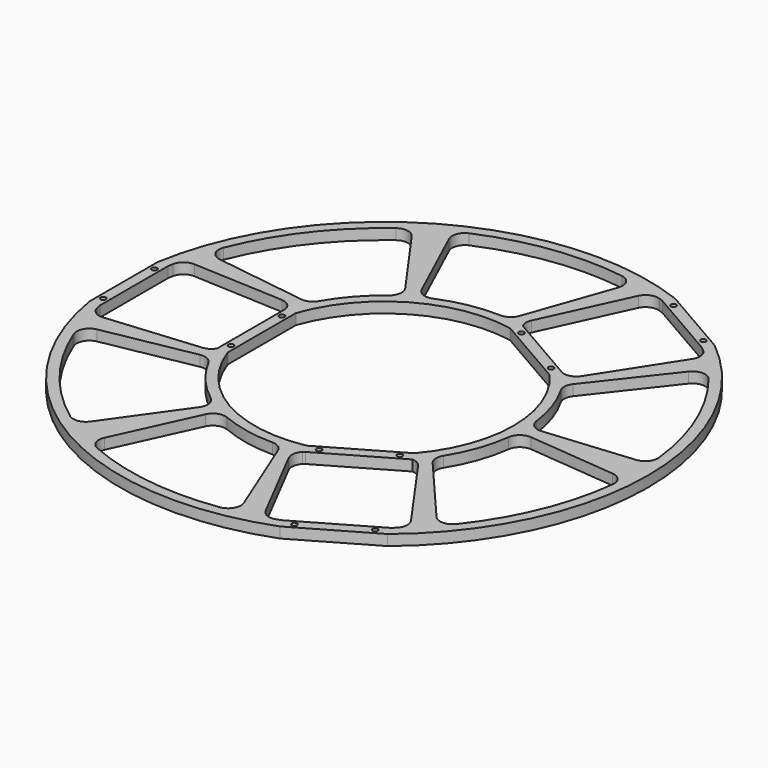
from build123d import *

# Parameters (mm, degrees)
F0_W        = 6.35
F0_H        = 50.8
F0_R        = 1.5875
F1_DEPTH    = 6.35
F4_DEPTH    = 6.35
F5_T1_DEPTH = 6.35
F6_R        = 5.08
F7_COUNT    = 3


# Not quite as in the source:
# - a fillet or chamfer that OpenCascade refuses, or shapes differently, is made with other operations: its cross-section is extruded or revolved along the edge and cut away or added
# - a feature of the source that left no trace in its solid (it failed there, or was rolled back) is left out


with BuildPart() as f1:
    # F0 (on Top) → F1 (new body)
    with BuildSketch(Plane.XY):
        with Locations((-76.2, 0)):
            Rectangle(F0_W, F0_H)
        with Locations((-76.2, -19.05)):
            Circle(F0_R, mode=Mode.SUBTRACT)
        with Locations((-76.2, 19.05)):
            Circle(F0_R, mode=Mode.SUBTRACT)
    extrude(amount=F1_DEPTH)



with BuildPart() as f1b:
    # F0 (on Top) → F1, piece 2 (new body)
    with BuildSketch(Plane.XY):
        with Locations((-152.4, 0)):
            Rectangle(F0_W, F0_H)
        with Locations((-152.4, -19.05)):
            Circle(F0_R, mode=Mode.SUBTRACT)
        with Locations((-152.4, 19.05)):
            Circle(F0_R, mode=Mode.SUBTRACT)
    extrude(amount=F1_DEPTH)


with BuildPart() as f1_1:
    add(f1.part)

    add(f1b.part)  # F4 merges F1b
    # F3 (on Top) → F4 (join)
    with BuildSketch(Plane.XY):
        with BuildLine():
            ThreePointArc((31.2797741547, 148.1041402319), (37.4651836805, 146.6615854162), (43.584633363, 144.9608235339))
            ThreePointArc((43.584633363, 144.9608235339), (48.1238684074, 143.5177825724), (52.6154547439, 141.9326408797))
            Line((52.6154547439, 141.9326408797), (55.7904547439, 147.4319021938))
            ThreePointArc((55.7904547439, 147.4319021938), (-78.8174165794, 136.5157700368), (-155.575, 25.4))
            Line((-155.575, 25.4), (-149.225, 25.4))
            ThreePointArc((-149.225, 25.4), (-148.3519798062, 30.0823987171), (-147.3320724153, 34.7350120599))
            ThreePointArc((-147.3320724153, 34.7350120599), (-145.7452505699, 40.8849918834), (-143.9018349238, 46.9629910733))
            ThreePointArc((-143.9018349238, 46.9629910733), (-120.5170928624, 91.5908890283), (-83.7806024253, 126.0716910423))
            ThreePointArc((-83.7806024253, 126.0716910423), (-75.6856337507, 131.0913630593), (-67.2909859281, 135.5919755658))
            ThreePointArc((-67.2909859281, 135.5919755658), (-19.0614902225, 150.1663085232), (31.2797741547, 148.1041402319))
        make_face()
        with BuildLine():
            ThreePointArc((8.2856324479, 82.9270698864), (11.4388872215, 82.551211282), (14.5755338083, 82.0554960938))
            Line((14.5755338083, 82.0554960938), (43.584633363, 144.9608235339))
            ThreePointArc((43.584633363, 144.9608235339), (37.4651836805, 146.6615854162), (31.2797741547, 148.1041402319))
            Line((31.2797741547, 148.1041402319), (8.2856324479, 82.9270698864))
        make_face()
        with BuildLine():
            ThreePointArc((-44.3888773768, 70.534943044), (-41.6699850762, 72.1745313026), (-38.8906138422, 73.7093669758))
            Line((-38.8906138422, 73.7093669758), (-67.2909859281, 135.5919755658))
            ThreePointArc((-67.2909859281, 135.5919755658), (-75.6856337507, 131.0913630593), (-83.7806024253, 126.0716910423))
            Line((-83.7806024253, 126.0716910423), (-44.3888773768, 70.534943044))
        make_face()
        with BuildLine():
            Line((-147.3320724153, 34.7350120599), (-77.2106727023, 31.3697728054))
            ThreePointArc((-77.2106727023, 31.3697728054), (-75.9595282254, 34.2884921917), (-74.5980976675, 37.1574279168))
            Line((-74.5980976675, 37.1574279168), (-143.9018349238, 46.9629910733))
            ThreePointArc((-143.9018349238, 46.9629910733), (-145.7452505699, 40.8849918834), (-147.3320724153, 34.7350120599))
        make_face()
        with BuildLine():
            ThreePointArc((-73.025, 25.4), (-38.6581512265, 66.957882051), (14.5154547439, 75.9415051114))
            Line((14.5154547439, 75.9415051114), (17.6904547439, 81.4407664254))
            ThreePointArc((17.6904547439, 81.4407664254), (16.1359219586, 81.762966235), (14.5755338083, 82.0554960938))
            ThreePointArc((14.5755338083, 82.0554960938), (11.4388872215, 82.551211282), (8.2856324479, 82.9270698864))
            ThreePointArc((8.2856324479, 82.9270698864), (-15.9814809475, 81.7932936843), (-38.8906138422, 73.7093669758))
            ThreePointArc((-38.8906138422, 73.7093669758), (-41.6699850762, 72.1745313026), (-44.3888773768, 70.534943044))
            ThreePointArc((-44.3888773768, 70.534943044), (-61.7898833675, 55.9246004763), (-74.5980976675, 37.1574279168))
            ThreePointArc((-74.5980976675, 37.1574279168), (-75.9595282254, 34.2884921917), (-77.2106727023, 31.3697728054))
            ThreePointArc((-77.2106727023, 31.3697728054), (-78.3497145543, 28.4055074635), (-79.375, 25.4))
            Line((-79.375, 25.4), (-73.025, 25.4))
        make_face()
    extrude(amount=F4_DEPTH)

    # F5: fillet of radius 7.62 on 12 edges, made by hand

    # F5_s2 → F5_t1 (join)
    with BuildSketch(Plane.XY):
        with BuildLine():
            ThreePointArc((-90.1475782146, 121.6004719031), (-84.410893045, 123.0042579182), (-79.3942694829, 119.8875834167))
            Line((-79.3942694829, 119.8875834167), (-83.7806024253, 126.0716910423))
            ThreePointArc((-83.7806024253, 126.0716910423), (-86.9928212861, 123.8769941098), (-90.1475782146, 121.6004719031))
        make_face()
        with BuildLine():
            ThreePointArc((-134.6146538369, 45.648977655), (-140.1386521152, 49.370669263), (-140.6262545751, 56.0135443368))
            ThreePointArc((-140.6262545751, 56.0135443368), (-142.3359988094, 51.5143093511), (-143.9018349238, 46.9629910733))
            Line((-143.9018349238, 46.9629910733), (-134.6146538369, 45.648977655))
        make_face()
        with BuildLine():
            ThreePointArc((-79.8602845165, 37.90195783), (-75.4541334055, 38.5971573414), (-72.1920699233, 41.6395925194))
            ThreePointArc((-72.1920699233, 41.6395925194), (-73.4292909895, 39.4168726535), (-74.5980976675, 37.1574279168))
            Line((-74.5980976675, 37.1574279168), (-79.8602845165, 37.90195783))
        make_face()
        with BuildLine():
            ThreePointArc((-48.8418760227, 76.8130398608), (-47.5248753854, 71.2518102655), (-50.4448624125, 66.3390268333))
            ThreePointArc((-50.4448624125, 66.3390268333), (-47.463259252, 68.50393891), (-44.3888773768, 70.534943044))
            Line((-44.3888773768, 70.534943044), (-48.8418760227, 76.8130398608))
        make_face()
        with BuildLine():
            ThreePointArc((-32.2288512937, 76.8560457563), (-37.9434400628, 76.7836545282), (-42.10110585, 80.7048253346))
            Line((-42.10110585, 80.7048253346), (-38.8906138422, 73.7093669758))
            ThreePointArc((-38.8906138422, 73.7093669758), (-35.5945217294, 75.3563577136), (-32.2288512937, 76.8560457563))
        make_face()
        with BuildLine():
            ThreePointArc((2.7684553264, 83.2939750529), (7.3191534676, 84.6172910948), (10.2074987686, 88.3746146557))
            Line((10.2074987686, 88.3746146557), (8.2856324479, 82.9270698864))
            ThreePointArc((8.2856324479, 82.9270698864), (5.5300876106, 83.1562911392), (2.7684553264, 83.2939750529))
        make_face()
        with BuildLine():
            ThreePointArc((22.2329863038, 149.7296061072), (27.6412349333, 146.1237556106), (28.2996981684, 139.6570920806))
            Line((28.2996981684, 139.6570920806), (31.2797741547, 148.1041402319))
            ThreePointArc((31.2797741547, 148.1041402319), (26.7687208847, 148.9855570423), (22.2329863038, 149.7296061072))
        make_face()
        with BuildLine():
            ThreePointArc((-64.1285580958, 128.7012459955), (-64.3193656083, 134.6041066922), (-60.2353086729, 138.870328775))
            ThreePointArc((-60.2353086729, 138.870328775), (-63.7842132005, 137.2764902356), (-67.2909859281, 135.5919755658))
            Line((-67.2909859281, 135.5919755658), (-64.1285580958, 128.7012459955))
        make_face()
        with BuildLine():
            ThreePointArc((-148.71471153, 28.234645377), (-145.9460574533, 32.7973396391), (-140.8631663364, 34.4245588066))
            Line((-140.8631663364, 34.4245588066), (-147.3320724153, 34.7350120599))
            ThreePointArc((-147.3320724153, 34.7350120599), (-148.0590701809, 31.4924175344), (-148.71471153, 28.234645377))
        make_face()
        with BuildLine():
            ThreePointArc((-86.5356054314, 31.8172913917), (-81.8153136869, 29.8806795078), (-79.375, 25.4))
            ThreePointArc((-79.375, 25.4), (-78.3497145543, 28.4055074635), (-77.2106727023, 31.3697728054))
            Line((-77.2106727023, 31.3697728054), (-86.5356054314, 31.8172913917))
        make_face()
        with BuildLine():
            ThreePointArc((40.7477165489, 138.8090579205), (44.6975181874, 142.6354540642), (50.194139768, 142.8068939441))
            ThreePointArc((50.194139768, 142.8068939441), (46.901752906, 143.9218058508), (43.584633363, 144.9608235339))
            Line((43.584633363, 144.9608235339), (40.7477165489, 138.8090579205))
        make_face()
        with BuildLine():
            ThreePointArc((17.6904547439, 81.4407664254), (16.7569695627, 84.8394313215), (17.4527300656, 88.294606423))
            Line((17.4527300656, 88.294606423), (14.5755338083, 82.0554960938))
            ThreePointArc((14.5755338083, 82.0554960938), (16.1359219586, 81.762966235), (17.6904547439, 81.4407664254))
        make_face()
    extrude(amount=F5_T1_DEPTH)

    # F6
    f6_edges = [f1_1.edges().sort_by_distance(p)[0] for p in [
        (-79.375, 25.4, 3.175),
    ]]
    fillet(f6_edges, radius=F6_R)

    # F7: F1 ×3 about axis
    f7_axis = Axis((0, 0, 0), (0, 0, 1))


with BuildPart() as f1_2:
    add(f1_1.part)
    for i in range(1, F7_COUNT):
        add(f1_1.part.rotate(f7_axis, i * 360 / F7_COUNT))


solid = f1_2.part
